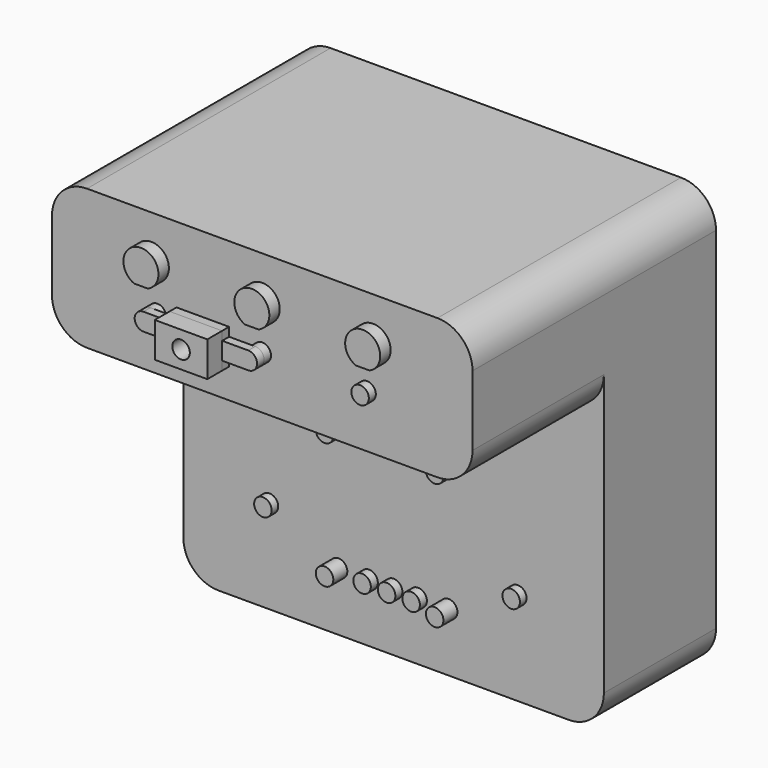
from build123d import *
from build123d import SkipClean  # not in build123d's __all__

# Parameters (mm, degrees)
F0_W      = 76.2
F0_H      = 38.1
F0_R      = 1.5875
F1_DEPTH  = 25.4
F2_R      = 1.5875
F3_DEPTH  = 1.5875
F4_R      = 1.5875
F5_DEPTH  = 31.34614
F6_W      = 76.2
F6_H      = 38.1
F7_DEPTH  = 29.75864
F8_R      = 1.5875
F9_DEPTH  = 1.5875
F10_R     = 1.5875
F11_DEPTH = 25.4
F12_W     = 76.2
F12_H     = 12.7
F13_DEPTH = 29.75864
F14_R     = 6.35
F16_DEPTH = 1.5748
F17_R     = 1.5875
F18_DEPTH = 4.9276
F19_R     = 1.5875
F20_DEPTH = 1.5875
F22_DEPTH = 2.3622
F23_R     = 1.5875
F24_DEPTH = 1.488


# Not quite as in the source:
# - a feature names something its author has since deleted; it is built from what else it names


with BuildPart() as f1:
    # F0 (on Front) → F1 (new body)
    with BuildSketch(Plane.XZ):
        with Locations((0, -19.05)):
            Rectangle(F0_W, F0_H)
        with Locations((-9.97712, -27.4772621454)):
            Circle(F0_R, mode=Mode.SUBTRACT)
        with Locations((-4.445, -27.4772621454)):
            Circle(F0_R, mode=Mode.SUBTRACT)
        with Locations((-9.97712, -4.6172621454)):
            Circle(F0_R, mode=Mode.SUBTRACT)
        with Locations((4.445, -27.4772621454)):
            Circle(F0_R, mode=Mode.SUBTRACT)
        with Locations((9.97712, -27.4772621454)):
            Circle(F0_R, mode=Mode.SUBTRACT)
        with Locations((9.97712, -4.6172621454)):
            Circle(F0_R, mode=Mode.SUBTRACT)
        with Locations((0, 19.05)):
            Rectangle(F0_W, F0_H)
        with Locations((-18.9992, 22.3118178546)):
            Circle(F0_R, mode=Mode.SUBTRACT)
        with Locations((0, 22.3118178546)):
            Circle(F0_R, mode=Mode.SUBTRACT)
        with Locations((18.9992, 22.3118178546)):
            Circle(F0_R, mode=Mode.SUBTRACT)
    extrude(amount=-F1_DEPTH)

    # F2 (on Front) → F3 (join)
    with BuildSketch(Plane.XZ):
        with Locations((9.97712, -4.6172621454)):
            Circle(F2_R)
        with Locations((-9.97712, -4.6172621454)):
            Circle(F2_R)
        with Locations((-9.97712, -27.4772621454)):
            Circle(F2_R)
        with Locations((-4.445, -27.4772621454)):
            Circle(F2_R)
        with Locations((4.445, -27.4772621454)):
            Circle(F2_R)
        with Locations((9.97712, -27.4772621454)):
            Circle(F2_R)
    extrude(amount=F3_DEPTH)

    # F4 (on Front) → F5 (join)
    with BuildSketch(Plane.XZ):
        with Locations((-18.9992, 22.3118178546)):
            Circle(F4_R)
        with Locations((0, 22.3118178546)):
            Circle(F4_R)
        with Locations((18.9992, 22.3118178546)):
            Circle(F4_R)
    extrude(amount=F5_DEPTH)

    # F6 (on Front) → F7 (join)
    with BuildSketch(Plane.XZ):
        with Locations((0, 19.05)):
            Rectangle(F6_W, F6_H)
    extrude(amount=F7_DEPTH)

    # F8 (on face) → F9 (join)
    with BuildSketch(Plane.XZ.offset(1.5875)):
        with Locations((-9.97712, -4.6172621454)):
            Circle(F8_R)
        with Locations((-9.97712, -27.4772621454)):
            Circle(F8_R)
        with Locations((9.97712, -27.4772621454)):
            Circle(F8_R)
        with Locations((9.97712, -4.6172621454)):
            Circle(F8_R)
    extrude(amount=F9_DEPTH)

    # F10 (on face) → F11 (join, through all)
    with BuildSketch(Plane(origin=(0, 25.4, 0), x_dir=(-1, 0, 0), z_dir=(0, 1, 0))):
        with Locations((9.97712, -27.4772621454)):
            Circle(F10_R)
        with Locations((4.445, -27.4772621454)):
            Circle(F10_R)
        with Locations((-4.445, -27.4772621454)):
            Circle(F10_R)
        with Locations((-9.97712, -27.4772621454)):
            Circle(F10_R)
        with Locations((9.97712, -4.6172621454)):
            Circle(F10_R)
        with Locations((-9.97712, -4.6172621454)):
            Circle(F10_R)
        with Locations((18.9992, 22.3118178546)):
            Circle(F10_R)
        with Locations((0, 22.3118178546)):
            Circle(F10_R)
        with Locations((-18.9992, 22.3118178546)):
            Circle(F10_R)
    extrude(amount=-F11_DEPTH)

    # F12 (on face) → F13 (cut, through all)
    with BuildSketch(Plane.XZ.offset(29.75864)):
        with Locations((0, 6.35)):
            Rectangle(F12_W, F12_H)
    extrude(amount=-F13_DEPTH, mode=Mode.SUBTRACT)

    # F14
    f14_edges = [f1.edges().sort_by_distance(p)[0] for p in [
        (-38.1, 12.7, -38.1),
        (38.1, 12.7, -38.1),
        (38.1, -14.87932, 12.7),
        (38.1, -2.17932, 38.1),
        (-38.1, -14.87932, 12.7),
        (-38.1, -2.17932, 38.1),
    ]]
    fillet(f14_edges, radius=F14_R)

    # F19 (on face) → F20 (join)
    with BuildSketch(Plane.XZ):
        with Locations((0, -27.4772621454)):
            Circle(F19_R)
    extrude(amount=F20_DEPTH)

    # F21 (on face) → F22 (join)
    with BuildSketch(Plane.XZ.offset(29.75864)):
        with BuildLine():
            ThreePointArc((21.3237476918, 27.3105378546), (20.0914, 33.4116178546), (18.8590523082, 27.3105378546))
            Line((18.8590523082, 27.3105378546), (21.3237476918, 27.3105378546))
        make_face()
        with BuildLine():
            Line((-21.3237476918, 27.3105378546), (-18.8590523082, 27.3105378546))
            ThreePointArc((-18.8590523082, 27.3105378546), (-20.0914, 33.4116178546), (-21.3237476918, 27.3105378546))
        make_face()
        with BuildLine():
            Line((-1.2323476918, 27.3105378546), (1.2323476918, 27.3105378546))
            ThreePointArc((1.2323476918, 27.3105378546), (0, 33.4116178546), (-1.2323476918, 27.3105378546))
        make_face()
    extrude(amount=F22_DEPTH)

    # F23 (on face) → F24 (join)
    with BuildSketch(Plane.XZ):
        with Locations((-22.4992, -21.1881821454)):
            Circle(F23_R)
        with Locations((22.4992, -21.1881821454)):
            Circle(F23_R)
    extrude(amount=F24_DEPTH)


with BuildPart() as f16:
    # F15 (on face) → F16 (new body)
    with BuildSketch(Plane.XZ.offset(31.34614)):
        with BuildLine():
            Line((-14.2621, 19.1368178546), (-9.4996, 19.1368178546))
            Line((-9.4996, 19.1368178546), (-9.4996, 20.7243178546))
            ThreePointArc((-9.4996, 20.7243178546), (-11.0871, 22.3118178546), (-9.4996, 23.8993178546))
            Line((-9.4996, 23.8993178546), (-9.4996, 25.4868178546))
            Line((-9.4996, 25.4868178546), (-14.2621, 25.4868178546))
            Line((-14.2621, 25.4868178546), (-14.2621, 23.8993178546))
            Line((-14.2621, 23.8993178546), (-18.9992, 23.8993178546))
            ThreePointArc((-18.9992, 23.8993178546), (-17.8766679849, 23.4343498698), (-17.4117, 22.3118178546))
            ThreePointArc((-17.4117, 22.3118178546), (-17.8766679849, 21.1892858395), (-18.9992, 20.7243178546))
            Line((-18.9992, 20.7243178546), (-14.2621, 20.7243178546))
            Line((-14.2621, 20.7243178546), (-14.2621, 19.1368178546))
        make_face()
        with BuildLine():
            Line((-4.7371, 20.7243178546), (0, 20.7243178546))
            ThreePointArc((0, 20.7243178546), (1.5875, 22.3118178546), (0, 23.8993178546))
            Line((0, 23.8993178546), (-4.7371, 23.8993178546))
            Line((-4.7371, 23.8993178546), (-4.7371, 25.4868178546))
            Line((-4.7371, 25.4868178546), (-9.4996, 25.4868178546))
            Line((-9.4996, 25.4868178546), (-9.4996, 23.8993178546))
            ThreePointArc((-9.4996, 23.8993178546), (-8.3770679849, 23.4343498698), (-7.9121, 22.3118178546))
            ThreePointArc((-7.9121, 22.3118178546), (-8.3770679849, 21.1892858395), (-9.4996, 20.7243178546))
            Line((-9.4996, 20.7243178546), (-9.4996, 19.1368178546))
            Line((-9.4996, 19.1368178546), (-4.7371, 19.1368178546))
            Line((-4.7371, 19.1368178546), (-4.7371, 20.7243178546))
        make_face()
        with BuildLine():
            ThreePointArc((-18.9992, 23.8993178546), (-20.5867, 22.3118178546), (-18.9992, 20.7243178546))
            ThreePointArc((-18.9992, 20.7243178546), (-17.8766679849, 21.1892858395), (-17.4117, 22.3118178546))
            ThreePointArc((-17.4117, 22.3118178546), (-17.8766679849, 23.4343498698), (-18.9992, 23.8993178546))
        make_face()
    extrude(amount=F16_DEPTH)

    # F17 (on face) → F18 (join)
    with BuildSketch(Plane.XZ.offset(31.34614)):
        Polygon((-4.7371, 23.8993178546), (-4.7371, 25.4868178546), (-14.2621, 25.4868178546), (-14.2621, 23.8993178546), (-14.2621, 20.7243178546), (-14.2621, 19.1368178546), (-4.7371, 19.1368178546), (-4.7371, 20.7243178546), align=None)
        with Locations((-9.4996, 22.3118178546)):
            Circle(F17_R, mode=Mode.SUBTRACT)
    with SkipClean():  # cleaning this boolean's faces spoils the solid; the shape is the same uncleaned
        extrude(amount=F18_DEPTH)


solid = Compound([f1.part, f16.part])
